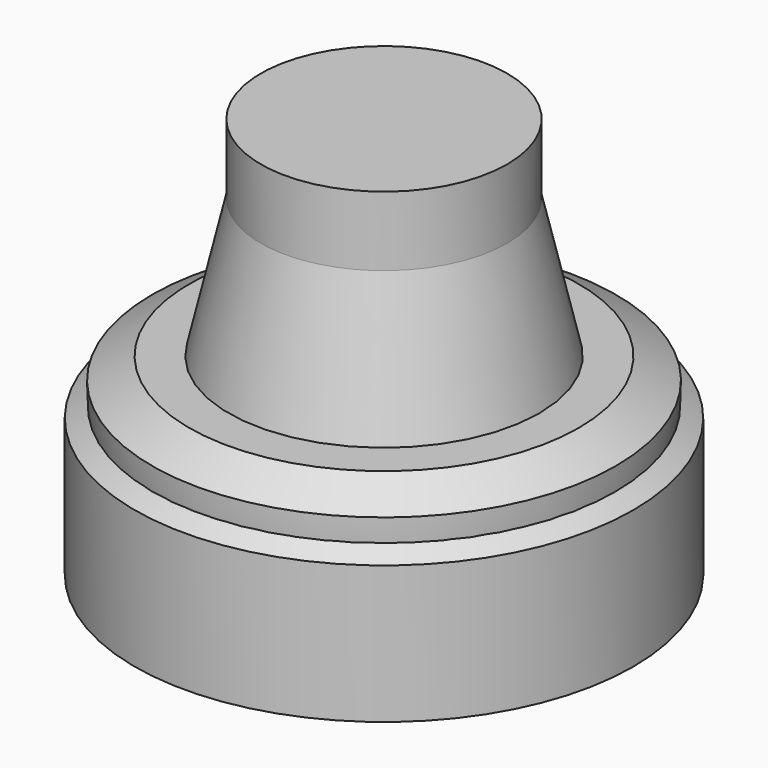
from build123d import *

# Parameters (mm, degrees)
F3_DEPTH = 7.5
F4_R     = 4.75


# Not quite as in the source:
# - an extrude ends at something that could not be found from the text; its depth is read off the source's solid
# - an extrude whose draft closes it to a point is written as a loft to that point


with BuildPart() as f1:
    # F0 (on Front) → F1 (revolve)
    with BuildSketch(Plane.XZ):
        with BuildLine():
            Line((8.4, 7.5), (4.6, 7.5))
            Line((4.6, 7.5), (4.6, 2.5))
            Line((4.6, 2.5), (1, 0.4215390309))
            Line((1, 0.4215390309), (0, 0.4215390309))
            Line((0, 0.4215390309), (0, 0))
            Line((0, 0), (8.4232673012, 0))
            ThreePointArc((8.4232673012, 0), (8.4841434441, 0.020664666), (8.5198598838, 0.0741180955))
            Line((8.5198598838, 0.0741180955), (8.5337299547, 0.1258819045))
            ThreePointArc((8.5337299547, 0.1258819045), (8.5694463944, 0.179335334), (8.6303225373, 0.2))
            Line((8.6303225373, 0.2), (10.75, 0.2))
            Line((10.75, 0.2), (10.75, 6.1432268674))
            Line((10.75, 6.1432268674), (8.4, 7.5))
        make_face()
    revolve(axis=Axis((0, 0, 0.2107695155), (0, 0, -1)))

    # F2 (on face) → F3 (join, through all)
    with BuildSketch(Plane.XY.offset(7.5)):
        with BuildLine():
            Line((2.328319946, 3.9672315573), (4.5998832843, 0.0327684427))
            ThreePointArc((4.5998832843, 0.0327684427), (3.9837168574, 2.3), (2.328319946, 3.9672315573))
        make_face()
        with BuildLine():
            ThreePointArc((2.2715633383, 4), (2.3, 3.9837168574), (2.328319946, 3.9672315573))
            Line((2.328319946, 3.9672315573), (2.3094010768, 4))
            Line((2.3094010768, 4), (2.2715633383, 4))
        make_face()
        with BuildLine():
            Line((-2.2715633383, 4), (2.2715633383, 4))
            ThreePointArc((2.2715633383, 4), (0, 4.6), (-2.2715633383, 4))
        make_face()
        with BuildLine():
            ThreePointArc((-2.328319946, 3.9672315573), (-2.3, 3.9837168574), (-2.2715633383, 4))
            Line((-2.2715633383, 4), (-2.3094010768, 4))
            Line((-2.3094010768, 4), (-2.328319946, 3.9672315573))
        make_face()
        with BuildLine():
            Line((-4.5998832843, 0.0327684427), (-2.328319946, 3.9672315573))
            ThreePointArc((-2.328319946, 3.9672315573), (-3.9837168574, 2.3), (-4.5998832843, 0.0327684427))
        make_face()
        with BuildLine():
            ThreePointArc((-4.5998832843, -0.0327684427), (-4.6, 0), (-4.5998832843, 0.0327684427))
            Line((-4.5998832843, 0.0327684427), (-4.6188021535, 0))
            Line((-4.6188021535, 0), (-4.5998832843, -0.0327684427))
        make_face()
        with BuildLine():
            ThreePointArc((-4.5998832843, -0.0327684427), (-3.9837168574, -2.3), (-2.328319946, -3.9672315573))
            Line((-2.328319946, -3.9672315573), (-4.5998832843, -0.0327684427))
        make_face()
        with BuildLine():
            Line((-2.3094010768, -4), (-2.2715633383, -4))
            ThreePointArc((-2.2715633383, -4), (-2.3, -3.9837168574), (-2.328319946, -3.9672315573))
            Line((-2.328319946, -3.9672315573), (-2.3094010768, -4))
        make_face()
        with BuildLine():
            ThreePointArc((-2.2715633383, -4), (0, -4.6), (2.2715633383, -4))
            Line((2.2715633383, -4), (-2.2715633383, -4))
        make_face()
        with BuildLine():
            Line((2.3094010768, -4), (2.328319946, -3.9672315573))
            ThreePointArc((2.328319946, -3.9672315573), (2.3, -3.9837168574), (2.2715633383, -4))
            Line((2.2715633383, -4), (2.3094010768, -4))
        make_face()
        with BuildLine():
            ThreePointArc((2.328319946, -3.9672315573), (3.9837168574, -2.3), (4.5998832843, -0.0327684427))
            Line((4.5998832843, -0.0327684427), (2.328319946, -3.9672315573))
        make_face()
        with BuildLine():
            ThreePointArc((4.5998832843, 0.0327684427), (4.599970821, 0.0163843253), (4.6, 0))
            ThreePointArc((4.6, 0), (4.599970821, -0.0163843253), (4.5998832843, -0.0327684427))
            Line((4.5998832843, -0.0327684427), (4.6188021535, 0))
            Line((4.6188021535, 0), (4.5998832843, 0.0327684427))
        make_face()
    extrude(amount=-F3_DEPTH)

    # F4 (on face) → F5 section 0
    with BuildSketch(Plane.XY.offset(7.5), mode=Mode.PRIVATE) as f5_s0:
        Circle(F4_R)
    loft([f5_s0.sketch, Vertex(0, 0, 6.6624468416)], ruled=True, mode=Mode.SUBTRACT)


with BuildPart() as f7:
    # F6 (on Front) → F7 (revolve)
    with BuildSketch(Plane.XZ):
        with BuildLine():
            Line((5.31, 17.5), (0, 17.5))
            Line((0, 17.5), (0, 0))
            Line((0, 0), (6.1432441735, 0))
            ThreePointArc((6.1432441735, 0), (7.7084604872, 0.7549707267), (8.0919843031, 2.4499021087))
            Line((8.0919843031, 2.4499021087), (5.31, 14.5))
            Line((5.31, 14.5), (5.31, 17.5))
        make_face()
    revolve(axis=Axis((0, 0, 8.75), (0, 0, -1)))


with BuildPart() as f9:
    # F8 (on Front) → F9 (revolve)
    with BuildSketch(Plane.XZ):
        with BuildLine():
            Line((0, 6.6236116251), (0, 0))
            Line((0, 0), (7.7227463564, 0))
            ThreePointArc((7.7227463564, 0), (8.3384078318, 0.2119892464), (8.6930420827, 0.7580781044))
            Line((8.6930420827, 0.7580781044), (9.6753940425, 4.6980766149))
            ThreePointArc((9.6753940425, 4.6980766149), (9.9328422492, 6.1264273905), (10, 7.5762395693))
            Line((10, 7.5762395693), (8.4, 8.5))
            Line((8.4, 8.5), (5.25, 8.5))
            Line((5.25, 8.5), (2, 6.6236116251))
            Line((2, 6.6236116251), (0, 6.6236116251))
        make_face()
    revolve(axis=Axis((0, 0, 3.3118058126), (0, 0, 1)))


solid = Compound([f1.part, f7.part, f9.part])
